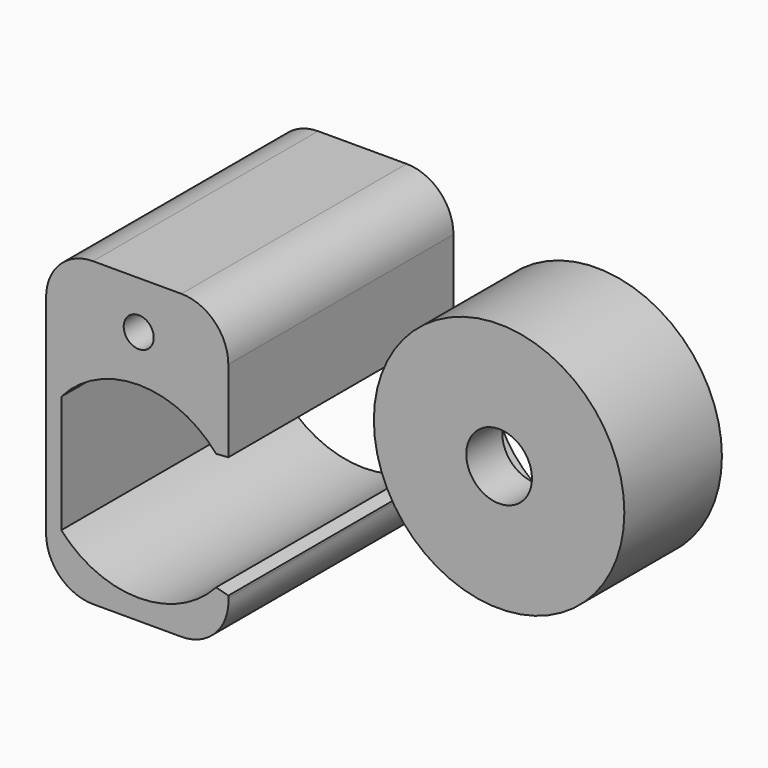
from build123d import *

# Parameters (mm, degrees)
F0_R     = 4.5755719827
F0_R_2   = 1.6
F1_DEPTH = 30
F2_R     = 13.35
F2_R_2   = 11.2454943051
F2_R_3   = 3.5
F3_DEPTH = 13
F4_DEPTH = 8.2
F5_DEPTH = 11.3


# Not quite as in the source:
# - a feature names something its author has since deleted; it is built from what else it names


with BuildPart() as f1:
    # F0 (on Front) → F1 (new body)
    with BuildSketch(Plane.XZ):
        with BuildLine():
            ThreePointArc((3.1984001178, -5.1894447684), (-5.0515998822, -8.8665109514), (-13.3015998822, -5.1894447684))
            Line((-13.3015998822, -5.1894447684), (-13.3015998822, 7.3447863489))
            ThreePointArc((-13.3015998822, 7.3447863489), (-5.0515998822, 11.1360002928), (3.1984001178, 7.3447863489))
            Line((3.1984001178, 7.3447863489), (4.4973706827, 7.4353506115))
            Line((4.4973706827, 7.4353506115), (4.4973706827, 16.1542760953))
            ThreePointArc((4.4973706827, 16.1542760953), (3.0329045886, 19.6898100013), (-0.5026293173, 21.1542760953))
            Line((-0.5026293173, 21.1542760953), (-9.9268148168, 21.1542760953))
            ThreePointArc((-9.9268148168, 21.1542760953), (-13.4623487228, 19.6898100013), (-14.9268148168, 16.1542760953))
            Line((-14.9268148168, 16.1542760953), (-14.9268148168, -6.0313575723))
            ThreePointArc((-14.9268148168, -6.0313575723), (-13.4623487228, -9.5668914783), (-9.9268148168, -11.0313575723))
            Line((-9.9268148168, -11.0313575723), (-0.4837697949, -11.0313575723))
            ThreePointArc((-0.4837697949, -11.0313575723), (3.1445739305, -9.4715787586), (4.5091521871, -5.7654062964))
            Line((4.5091521871, -5.7654062964), (4.4973706827, -5.5442224257))
            Line((4.4973706827, -5.5442224257), (3.1984001178, -5.1894447684))
        make_face()
        with Locations((-5.0515998822, 16.0776707903)):
            Circle(F0_R, mode=Mode.SUBTRACT)
        with Locations((-5.0515998822, 16.0776707903)):
            Circle(F0_R)
        with Locations((-5.0515998822, 16.0776707903)):
            Circle(F0_R_2, mode=Mode.SUBTRACT)
    extrude(amount=F1_DEPTH)

    # F0 (on Front) → F5 (cut)
    with BuildSketch(Plane.XZ):
        with Locations((-5.0515998822, 16.0776707903)):
            Circle(F0_R)
        with Locations((-5.0515998822, 16.0776707903)):
            Circle(F0_R_2, mode=Mode.SUBTRACT)
    extrude(amount=F5_DEPTH, mode=Mode.SUBTRACT)


with BuildPart() as f3:
    # F2 (on Front) → F3 (new body)
    with BuildSketch(Plane.XZ):
        with Locations((19.7629034519, 4.6483911574)):
            Circle(F2_R)
        with Locations((19.7629034519, 4.6483911574)):
            Circle(F2_R_2, mode=Mode.SUBTRACT)
        with Locations((19.7629034519, 4.6483911574)):
            Circle(F2_R_2)
        with Locations((19.7629034519, 4.6483911574)):
            Circle(F2_R_3, mode=Mode.SUBTRACT)
    extrude(amount=F3_DEPTH)

    # F2 (on Front) → F4 (cut)
    with BuildSketch(Plane.XZ):
        with Locations((19.7629034519, 4.6483911574)):
            Circle(F2_R_2)
        with Locations((19.7629034519, 4.6483911574)):
            Circle(F2_R_3, mode=Mode.SUBTRACT)
    extrude(amount=F4_DEPTH, mode=Mode.SUBTRACT)


solid = Compound([f1.part, f3.part])
